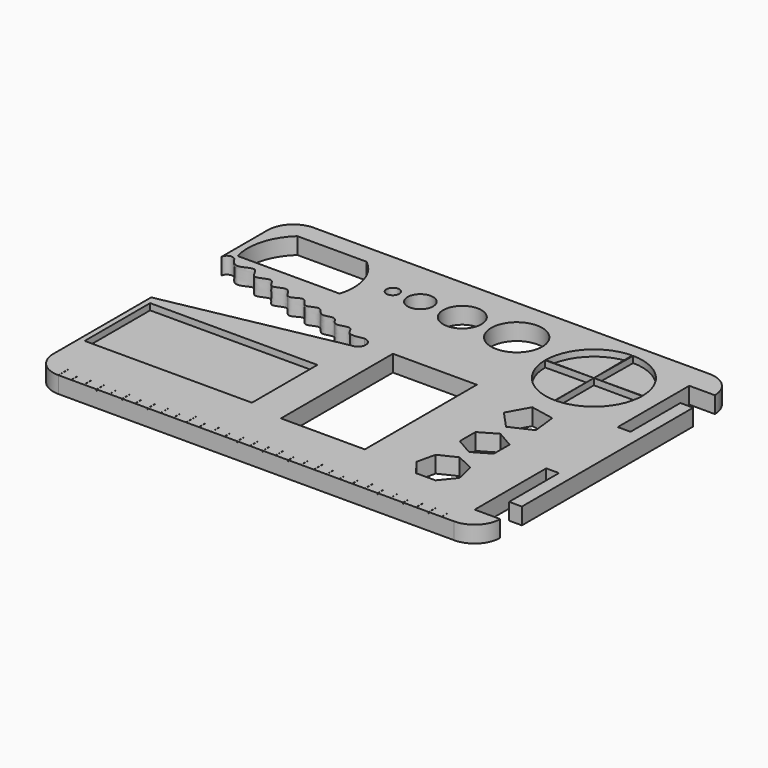
from build123d import *

# Parameters (mm, degrees)
F0_W      = 88.9
F0_H      = 63.5
F1_DEPTH  = 3.302
F3_R      = 5.08
F2_W      = 0.0254
F2_H      = 1.8163701752
F2_W_2    = 0.0299101812
F2_H_2    = 2.4313437752
F4_DEPTH  = 0.254
F5_R      = 1.27
F5_R_2    = 2.54
F5_R_3    = 3.81
F5_R_4    = 5.08
F6_DEPTH  = 25.4
F7_W      = 53.34
F7_H      = 3.302
F8_DEPTH  = 5.08
F9_W      = 17.78
F9_H      = 3.302
F10_DEPTH = 2.54
F12_DEPTH = 25.4
F14_DEPTH = 1.27
F16_DEPTH = 1.27
F17_W     = 16.6861191392
F17_H     = 27.8427181765
F18_DEPTH = 25.4
F19_W     = 33.2703352906
F19_H     = 16.2781784311
F20_DEPTH = 1.27
F22_DEPTH = 2.54


# Not quite as in the source:
# - ends of sketch curves that miss each other by under 0.0002 mm in the source are joined


with BuildPart() as f1:
    # F0 (on Top) → F1 (new body)
    with BuildSketch(Plane.XY):
        with Locations((44.45, 31.75)):
            Rectangle(F0_W, F0_H)
    extrude(amount=F1_DEPTH)

    # F3
    f3_edges = [f1.edges().sort_by_distance(p)[0] for p in [
        (0, 0, 1.651),
        (88.9, 0, 1.651),
        (88.9, 63.5, 1.651),
        (0, 63.5, 1.651),
    ]]
    fillet(f3_edges, radius=F3_R)

    # F2 (on face) → F4 (cut)
    with BuildSketch(Plane.XY.offset(3.302)):
        with Locations((81.2972101812, 0.9081850876)):
            Rectangle(F2_W, F2_H)
        with Locations((78.7572101812, 0.9081850876)):
            Rectangle(F2_W, F2_H)
        with Locations((76.2172101812, 0.9081850876)):
            Rectangle(F2_W, F2_H)
        with Locations((73.6772101812, 0.9081850876)):
            Rectangle(F2_W, F2_H)
        with Locations((71.1372101812, 0.9081850876)):
            Rectangle(F2_W, F2_H)
        with Locations((68.5972101812, 0.9081850876)):
            Rectangle(F2_W, F2_H)
        with Locations((66.0572101812, 0.9081850876)):
            Rectangle(F2_W, F2_H)
        with Locations((63.5172101812, 0.9081850876)):
            Rectangle(F2_W, F2_H)
        with Locations((60.9772101812, 0.9081850876)):
            Rectangle(F2_W, F2_H)
        with Locations((58.4372101812, 0.9081850876)):
            Rectangle(F2_W, F2_H)
        Polygon((55.88, 2.4313437752), (55.88, 0), (55.9099101812, 0), (55.9099101812, 1.8163701752), (55.9099101812, 2.4313437752), align=None)
        with Locations((53.3572101812, 0.9081850876)):
            Rectangle(F2_W, F2_H)
        with Locations((50.8172101812, 0.9081850876)):
            Rectangle(F2_W, F2_H)
        with Locations((48.2772101812, 0.9081850876)):
            Rectangle(F2_W, F2_H)
        with Locations((45.7372101812, 0.9081850876)):
            Rectangle(F2_W, F2_H)
        with Locations((43.1972101812, 0.9081850876)):
            Rectangle(F2_W, F2_H)
        with Locations((40.6572101812, 0.9081850876)):
            Rectangle(F2_W, F2_H)
        with Locations((38.1172101812, 0.9081850876)):
            Rectangle(F2_W, F2_H)
        with Locations((35.5772101812, 0.9081850876)):
            Rectangle(F2_W, F2_H)
        with Locations((33.0372101812, 0.9081850876)):
            Rectangle(F2_W, F2_H)
        Polygon((30.48, 2.4313437752), (30.48, 0), (30.5099101812, 0), (30.5099101812, 1.8163701752), (30.5099101812, 2.4313437752), align=None)
        with Locations((27.9572101812, 0.9081850876)):
            Rectangle(F2_W, F2_H)
        with Locations((25.4172101812, 0.9081850876)):
            Rectangle(F2_W, F2_H)
        with Locations((22.8772101812, 0.9081850876)):
            Rectangle(F2_W, F2_H)
        with Locations((20.3372101812, 0.9081850876)):
            Rectangle(F2_W, F2_H)
        with Locations((17.7972101812, 0.9081850876)):
            Rectangle(F2_W, F2_H)
        with Locations((15.2572101812, 0.9081850876)):
            Rectangle(F2_W, F2_H)
        with Locations((12.7172101812, 0.9081850876)):
            Rectangle(F2_W, F2_H)
        with Locations((10.1772101812, 0.9081850876)):
            Rectangle(F2_W, F2_H)
        with Locations((7.6372101812, 0.9081850876)):
            Rectangle(F2_W, F2_H)
        with Locations((5.0949550906, 1.2156718876)):
            Rectangle(F2_W_2, F2_H_2)
        with BuildLine():
            Line((18.6525154859, 59.6915856004), (4.8563710406, 59.6915856004))
            ThreePointArc((4.8563710406, 59.6915856004), (1.7675174689, 54.628236872), (1.7819992009, 48.6971065402))
            Line((1.7819992009, 48.6971065402), (22.0637402854, 48.6971065402))
            ThreePointArc((22.0637402854, 48.6971065402), (22.0513701135, 54.7197033744), (18.6525154859, 59.6915856004))
        make_face()
    extrude(amount=-F4_DEPTH, mode=Mode.SUBTRACT)

    # F5 (on face) → F6 (cut)
    with BuildSketch(Plane.XY.offset(3.302)):
        with Locations((28.073919937, 54.4169172645)):
            Circle(F5_R)
        with Locations((33.5413217545, 54.4169172645)):
            Circle(F5_R_2)
        with Locations((41.886460036, 54.4169172645)):
            Circle(F5_R_3)
        with Locations((52.7133606374, 54.4169172645)):
            Circle(F5_R_4)
        with BuildLine():
            Line((18.6525154859, 59.6915856004), (4.8563710406, 59.6915856004))
            ThreePointArc((4.8563710406, 59.6915856004), (1.7675174689, 54.628236872), (1.7819992009, 48.6971065402))
            Line((1.7819992009, 48.6971065402), (22.0637402854, 48.6971065402))
            ThreePointArc((22.0637402854, 48.6971065402), (22.0513701135, 54.7197033744), (18.6525154859, 59.6915856004))
        make_face()
    extrude(amount=-F6_DEPTH, mode=Mode.SUBTRACT)

    # F7 (on face) → F8 (cut)
    with BuildSketch(Plane.YZ.offset(88.9)):
        with Locations((31.75, 1.651)):
            Rectangle(F7_W, F7_H)
    extrude(amount=-F8_DEPTH, mode=Mode.SUBTRACT)

    # F9 (on face) → F10 (join)
    with BuildSketch(Plane.YZ.offset(83.82)):
        with Locations((31.75, 1.651)):
            Rectangle(F9_W, F9_H)
    extrude(amount=F10_DEPTH)

    # F11 (on face) → F12 (cut)
    with BuildSketch(Plane.XY.offset(3.302)):
        with BuildLine():
            Line((0, 29.4399894774), (34.4703271985, 36.2297259271))
            ThreePointArc((34.4703271985, 36.2297259271), (36.0134504735, 37.7728492022), (34.4703271985, 39.3159724772))
            add(Edge.make_bspline(
                [(34.4703271985, 39.3159724772), (33.3339544716, 39.0753649595), (31.302492593, 38.6452376005), (30.8254271258, 41.5083466768), (27.6063276919, 39.4881789644), (26.8072303924, 42.5700243888), (24.0352227889, 40.6423937111), (22.9011599207, 43.8129110638), (20.1525319163, 41.2602511151), (19.0670906626, 44.8684872735), (16.2237788201, 41.7726497646), (15.1133816839, 45.8835126733), (11.9041477706, 43.0415205501), (11.2936256205, 46.7314166473), (7.757319112, 43.7208497558), (7.0863793612, 48.0076276779), (3.6989716146, 45.14915258), (2.5245619264, 46.8414412054), (1.9540779758, 47.6634912193)],
                knots=[0, 0, 0, 0, 0.0688507244, 0.1230825227, 0.1877804451, 0.2450114273, 0.3055063893, 0.3648925502, 0.4266471395, 0.4865115595, 0.5495998779, 0.6134740855, 0.6785906019, 0.7359414812, 0.8037454041, 0.8664475923, 0.9351252754, 1, 1, 1, 1], degree=3))
            ThreePointArc((1.9540779758, 47.6634912193), (0.7654634509, 47.9053844441), (0, 46.9644367695))
            Line((0, 46.9644367695), (0, 29.4399894774))
        make_face()
    extrude(amount=-F12_DEPTH, mode=Mode.SUBTRACT)

    # F13 (on face) → F14 (cut)
    with BuildSketch(Plane.XY.offset(3.302)):
        with BuildLine():
            ThreePointArc((80.2671810997, 51.1491746361), (80.2673034504, 51.177214745), (80.267344234, 51.2052550912))
            ThreePointArc((80.267344234, 51.2052550912), (80.2672966172, 51.2355535331), (80.2671537673, 51.2658516756))
            Line((80.2671537673, 51.2658516756), (70.627912879, 51.2052550912))
            Line((70.627912879, 51.2052550912), (80.2671810997, 51.1491746361))
        make_face()
        with BuildLine():
            Line((70.627912879, 51.2052550912), (80.2671537673, 51.2658516756))
            ThreePointArc((80.2671537673, 51.2658516756), (77.4592351409, 58.0061133461), (70.7315905113, 60.8441288738))
            Line((70.7315905113, 60.8441288738), (70.627912879, 51.2052550912))
        make_face()
        with BuildLine():
            ThreePointArc((70.6644242274, 41.5658928836), (77.4370978416, 44.382232521), (80.2671810997, 51.1491746361))
            Line((80.2671810997, 51.1491746361), (70.627912879, 51.2052550912))
            Line((70.627912879, 51.2052550912), (70.6644242274, 41.5658928836))
        make_face()
        with BuildLine():
            Line((70.627912879, 51.2052550912), (70.7315905113, 60.8441288738))
            ThreePointArc((70.7315905113, 60.8441288738), (70.6318533156, 60.8446856408), (70.532115698, 60.8442104157))
            Line((70.532115698, 60.8442104157), (70.627912879, 51.2052550912))
        make_face()
        with BuildLine():
            Line((60.9887407095, 51.2759426865), (70.627912879, 51.2052550912))
            Line((70.627912879, 51.2052550912), (70.532115698, 60.8442104157))
            ThreePointArc((70.532115698, 60.8442104157), (63.8029334726, 58.0124786772), (60.9887407095, 51.2759426865))
        make_face()
        with BuildLine():
            Line((70.6644242274, 41.5658928836), (70.627912879, 51.2052550912))
            Line((70.627912879, 51.2052550912), (70.5950788503, 41.5658796563))
            ThreePointArc((70.5950788503, 41.5658796563), (70.6297515507, 41.5658239115), (70.6644242274, 41.5658928836))
        make_face()
        with BuildLine():
            Line((60.9886712858, 51.1447707469), (70.627912879, 51.2052550912))
            Line((70.627912879, 51.2052550912), (60.9887407095, 51.2759426865))
            ThreePointArc((60.9887407095, 51.2759426865), (60.988482874, 51.2103568348), (60.9886712858, 51.1447707469))
        make_face()
        with BuildLine():
            Line((70.5950788503, 41.5658796563), (70.627912879, 51.2052550912))
            Line((70.627912879, 51.2052550912), (60.9886712858, 51.1447707469))
            ThreePointArc((60.9886712858, 51.1447707469), (63.821588589, 44.3793788465), (70.5950788503, 41.5658796563))
        make_face()
    extrude(amount=-F14_DEPTH, mode=Mode.SUBTRACT)

    # F17 (on face) → F18 (cut)
    with BuildSketch(Plane.XY.offset(3.302)):
        with Locations((49.4981966913, 24.1656512953)):
            Rectangle(F17_W, F17_H)
        Polygon((70.2164718428, 29.8823021758), (74.5598822832, 31.8874642253), (73.9950474894, 36.6379221774), (69.3025499484, 37.5687046044), (66.9672617697, 33.3935018283), align=None)
        Polygon((74.3968502494, 25.5366461352), (71.0082426667, 27.4930596352), (67.6196350841, 25.5366461352), (67.6196350841, 21.6238191351), (71.0082426667, 19.6674056351), (74.3968502494, 21.6238191351), align=None)
        Polygon((74.463043767, 15.6978405279), (71.0082426667, 17.3615850508), (67.5534415664, 15.6978405279), (66.7001761597, 11.959440519), (69.0909727014, 8.9614764804), (72.9255126321, 8.9614764804), (75.3163091737, 11.959440519), align=None)
    extrude(amount=-F18_DEPTH, mode=Mode.SUBTRACT)

    # F19 (on face) → F20 (cut)
    with BuildSketch(Plane.XY.offset(3.302)):
        with Locations((17.7104144823, 19.6877508424)):
            Rectangle(F19_W, F19_H)
    extrude(amount=-F20_DEPTH, mode=Mode.SUBTRACT)

    # F21 (on face) → F22 (join)
    with BuildSketch(Plane.YZ.offset(86.36)):
        Polygon((40.64, 3.302), (22.86, 3.302), (10.4681262746, 3.302), (10.4681262746, 0), (22.86, 0), (40.64, 0), (53.0352, 0), (53.0352, 3.302), align=None)
    extrude(amount=F22_DEPTH)


with BuildPart() as f16:
    # F15 (on face) → F16 (new body)
    with BuildSketch(Plane.XY.offset(2.032)):
        Polygon((70.5323335428, 60.8222912312), (70.627912879, 51.2052550912), (70.7313768992, 60.8242694324), align=None)
        Polygon((70.532115698, 60.8442104157), (70.5323335428, 60.8222912312), (70.7313768992, 60.8242694324), (70.7315905113, 60.8441288738), align=None)
    extrude(amount=F16_DEPTH)


with BuildPart() as f16b:
    # F15 (on face) → F16, piece 2 (new body)
    with BuildSketch(Plane.XY.offset(2.032)):
        Polygon((80.2577985466, 51.2657928645), (70.627912879, 51.2052550912), (80.2577985466, 51.149229223), align=None)
    extrude(amount=F16_DEPTH)


with BuildPart() as f16c:
    # F15 (on face) → F16, piece 3 (new body)
    with BuildSketch(Plane.XY.offset(2.032)):
        Polygon((61.0020025449, 51.144854398), (70.627912879, 51.2052550912), (61.0020030698, 51.2758454288), align=None)
    extrude(amount=F16_DEPTH)


with BuildPart() as f16d:
    # F15 (on face) → F16, piece 4 (new body)
    with BuildSketch(Plane.XY.offset(2.032)):
        Polygon((70.664391697, 41.5744812252), (70.627912879, 51.2052550912), (70.595108954, 41.5747174529), align=None)
    extrude(amount=F16_DEPTH)


solid = Compound([f1.part, f16.part, f16b.part, f16c.part, f16d.part])
